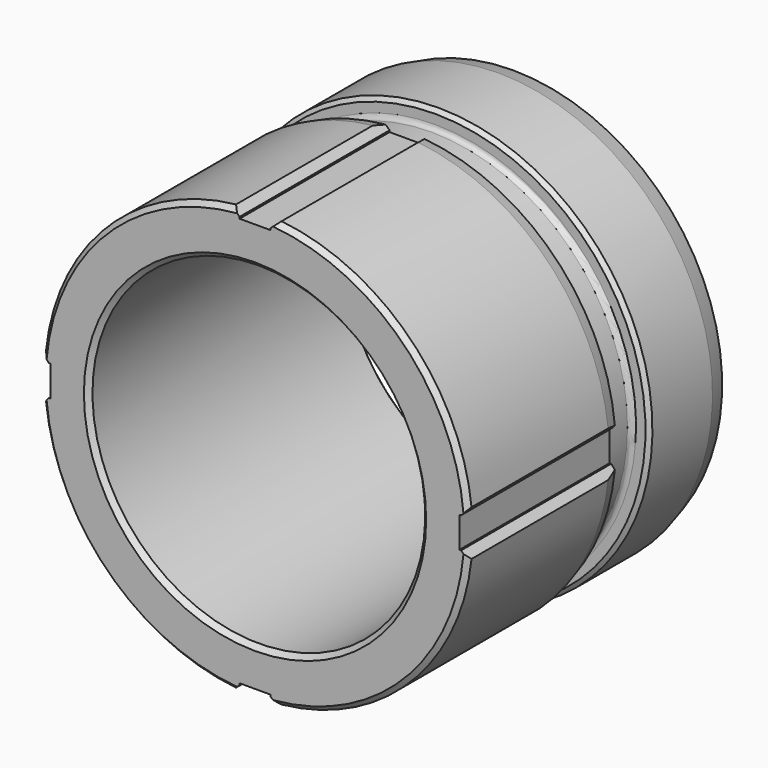
from build123d import *

# Parameters (mm, degrees)
F0_W            = 67.945
F0_H            = 10.0203
F2_SIZE         = 1
F3_SIZE2        = 1.0208864232
F3_SIZE         = 3.81
F4_W            = 8
F4_H            = 9.8567151233
F7_DEPTH        = 40
F7_COPIES_COUNT = 4
F8_T1_DEPTH     = 46.4577782779
F9_R            = 1
F10_SIZE        = 0.8128
F11_SIZE2       = 2.54
F11_SIZE        = 0.6805909488


# Not quite as in the source:
# - a fillet or chamfer that OpenCascade refuses, or shapes differently, is made with other operations: its cross-section is extruded or revolved along the edge and cut away or added
# - a pattern or mirror of a feature is missing from the dataset's text; its kind, count and spacing are read off the source's solid


with BuildPart() as f1:
    # F0 (on Right) → F1 (revolve)
    with BuildSketch(Plane.YZ):
        with Locations((33.9725, 40.06215)):
            Rectangle(F0_W, F0_H)
    revolve(axis=Axis((0, 10.0695292601, 0), (0, 1, 0)))

    # F2
    f2_edges = [f1.edges().sort_by_distance(p)[0] for p in [
        (0, 0, -35.052),
        (0, 0, -45.0723),
        (0, 67.945, -35.052),
    ]]
    chamfer(f2_edges, length=F2_SIZE)

    # F3
    f3_edges = [f1.edges().sort_by_distance(p)[0] for p in [
        (0, 67.945, -45.0723),
    ]]
    chamfer(f3_edges, length=F3_SIZE, length2=F3_SIZE2)

    # F4 (on Right) → F5 (revolve, cut)
    with BuildSketch(Plane.YZ):
        with Locations((43.5, 46.2033575617)):
            Rectangle(F4_W, F4_H)
    revolve(axis=Axis((0, 33.4974332383, 0), (0, 1, 0)), mode=Mode.SUBTRACT)

    # F6 (on face) → F7 (cut)
    with BuildSketch(Plane.XZ):
        Polygon((3.25, 49.6761292126), (0, 49.6761292126), (-3.25, 49.6761292126), (-3.25, 43.0723), (0, 43.0723), (3.25, 43.0723), align=None)
    f7 = extrude(amount=-F7_DEPTH, mode=Mode.SUBTRACT)

    # F7_copies: F7 ×4 about axis
    f7_copies_axis = Axis((0, 0, 0), (0, 1, 0))
    for i in range(1, F7_COPIES_COUNT):
        add(f7.rotate(f7_copies_axis, i * 360 / F7_COPIES_COUNT), mode=Mode.SUBTRACT)

    # F8: chamfer of 1.5 on 8 edges, made by hand

    # F8_s2 → F8_t1 (cut)
    with BuildSketch(Plane.XZ.offset(-43.478889139)):
        with BuildLine():
            Line((-4.8385212577, 44.8567419714), (-3.2053743546, 43.3889711075))
            Line((-3.2053743546, 43.3889711075), (-3.1753743546, 43.3889711075))
            ThreePointArc((-3.1753743546, 43.3889711075), (-3.22, 44.1719727759), (-3.22, 44.9549744443))
            Line((-3.22, 44.9549744443), (-3.2521631911, 44.9848963528))
            ThreePointArc((-3.2521631911, 44.9848963528), (-4.0455787179, 44.9204937431), (-4.8417120615, 44.8865718016))
            Line((-4.8417120615, 44.8865718016), (-4.8385212577, 44.8567419714))
        make_face()
        with BuildLine():
            Line((4.8385212577, 44.8567419714), (3.2053743546, 43.3889711075))
            Line((3.2053743546, 43.3889711075), (3.1753743546, 43.3889711075))
            ThreePointArc((3.1753743546, 43.3889711075), (3.22, 44.1719727759), (3.22, 44.9549744443))
            Line((3.22, 44.9549744443), (3.2521631911, 44.9848963528))
            ThreePointArc((3.2521631911, 44.9848963528), (4.0455787179, 44.9204937431), (4.8417120615, 44.8865718016))
            Line((4.8417120615, 44.8865718016), (4.8385212577, 44.8567419714))
        make_face()
        with BuildLine():
            Line((-44.8567419714, 4.8385212577), (-43.3889711075, 3.2053743546))
            Line((-43.3889711075, 3.2053743546), (-43.3889711075, 3.1753743546))
            ThreePointArc((-43.3889711075, 3.1753743546), (-44.1719727759, 3.22), (-44.9549744443, 3.22))
            Line((-44.9549744443, 3.22), (-44.9848963528, 3.2521631911))
            ThreePointArc((-44.9848963528, 3.2521631911), (-44.9204937431, 4.0455787179), (-44.8865718016, 4.8417120615))
            Line((-44.8865718016, 4.8417120615), (-44.8567419714, 4.8385212577))
        make_face()
        with BuildLine():
            Line((-43.3889711075, -3.2053743546), (-44.8567419714, -4.8385212577))
            Line((-44.8567419714, -4.8385212577), (-44.8865718016, -4.8417120615))
            ThreePointArc((-44.8865718016, -4.8417120615), (-44.9204937431, -4.0455787179), (-44.9848963528, -3.2521631911))
            Line((-44.9848963528, -3.2521631911), (-44.9549744443, -3.22))
            ThreePointArc((-44.9549744443, -3.22), (-44.1719727759, -3.22), (-43.3889711075, -3.1753743546))
            Line((-43.3889711075, -3.1753743546), (-43.3889711075, -3.2053743546))
        make_face()
        with BuildLine():
            Line((-4.8385212577, -44.8567419714), (-3.2053743546, -43.3889711075))
            Line((-3.2053743546, -43.3889711075), (-3.1753743546, -43.3889711075))
            ThreePointArc((-3.1753743546, -43.3889711075), (-3.22, -44.1719727759), (-3.22, -44.9549744443))
            Line((-3.22, -44.9549744443), (-3.2521631911, -44.9848963528))
            ThreePointArc((-3.2521631911, -44.9848963528), (-4.0455787179, -44.9204937431), (-4.8417120615, -44.8865718016))
            Line((-4.8417120615, -44.8865718016), (-4.8385212577, -44.8567419714))
        make_face()
        with BuildLine():
            Line((3.2053743546, -43.3889711075), (4.8385212577, -44.8567419714))
            Line((4.8385212577, -44.8567419714), (4.8417120615, -44.8865718016))
            ThreePointArc((4.8417120615, -44.8865718016), (4.0455787179, -44.9204937431), (3.2521631911, -44.9848963528))
            Line((3.2521631911, -44.9848963528), (3.22, -44.9549744443))
            ThreePointArc((3.22, -44.9549744443), (3.22, -44.1719727759), (3.1753743546, -43.3889711075))
            Line((3.1753743546, -43.3889711075), (3.2053743546, -43.3889711075))
        make_face()
        with BuildLine():
            Line((44.8567419714, -4.8385212577), (43.3889711075, -3.2053743546))
            Line((43.3889711075, -3.2053743546), (43.3889711075, -3.1753743546))
            ThreePointArc((43.3889711075, -3.1753743546), (44.1719727759, -3.22), (44.9549744443, -3.22))
            Line((44.9549744443, -3.22), (44.9848963528, -3.2521631911))
            ThreePointArc((44.9848963528, -3.2521631911), (44.9204937431, -4.0455787179), (44.8865718016, -4.8417120615))
            Line((44.8865718016, -4.8417120615), (44.8567419714, -4.8385212577))
        make_face()
        with BuildLine():
            Line((43.3889711075, 3.2053743546), (44.8567419714, 4.8385212577))
            Line((44.8567419714, 4.8385212577), (44.8865718016, 4.8417120615))
            ThreePointArc((44.8865718016, 4.8417120615), (44.9204937431, 4.0455787179), (44.9848963528, 3.2521631911))
            Line((44.9848963528, 3.2521631911), (44.9549744443, 3.22))
            ThreePointArc((44.9549744443, 3.22), (44.1719727759, 3.22), (43.3889711075, 3.1753743546))
            Line((43.3889711075, 3.1753743546), (43.3889711075, 3.2053743546))
        make_face()
    extrude(amount=F8_T1_DEPTH, mode=Mode.SUBTRACT)

    # F9
    f9_edges = [f1.edges().sort_by_distance(p)[0] for p in [
        (0, 39.5, -41.275),
        (0, 47.5, -41.275),
    ]]
    fillet(f9_edges, radius=F9_R)

    # F10
    f10_edges = [f1.edges().sort_by_distance(p)[0] for p in [
        (0, 47.5, -45.0723),
    ]]
    chamfer(f10_edges, length=F10_SIZE)

    # F11
    f11_edges = [f1.edges().sort_by_distance(p)[0] for p in [
        (-31.870929, 39.5, 31.870929),
        (-31.870929, 39.5, -31.870929),
        (31.870929, 39.5, -31.870929),
        (31.870929, 39.5, 31.870929),
    ]]
    f11_side = f1.faces().sort_by_distance((0, 39.5, -42.401761))[0]
    chamfer(f11_edges, length=F11_SIZE, length2=F11_SIZE2, reference=f11_side)


solid = f1.part
